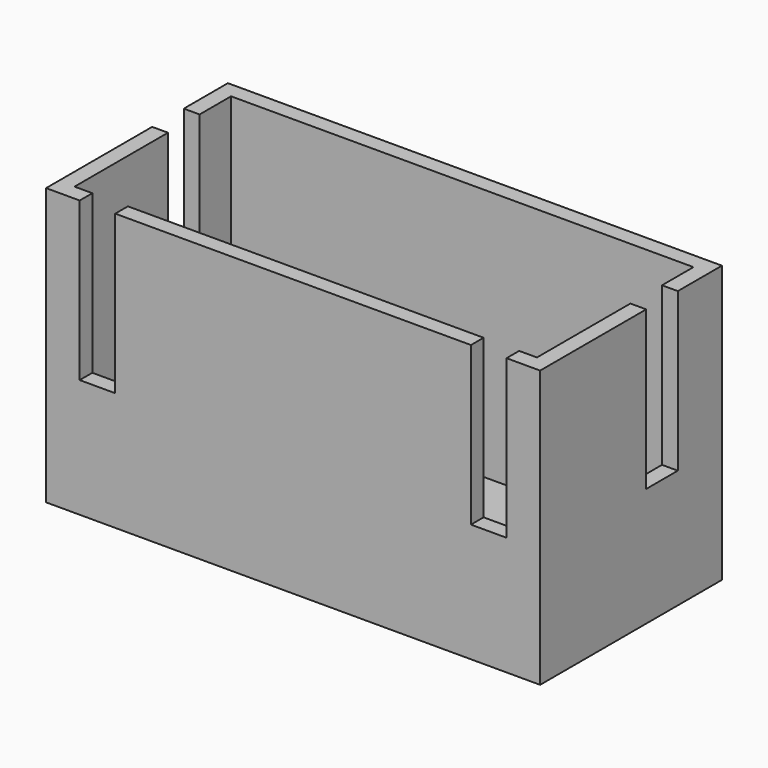
from build123d import *

# Parameters (mm, degrees)
F1_W      = 12.5
F1_H      = 5.75
F2_DEPTH  = 7
F3_W      = 11.7
F3_H      = 4.95
F4_DEPTH  = 6.4
F5_W      = 0.64
F5_H      = 0.64
F6_DEPTH  = 0.601
F7_W      = 0.9
F7_H      = 0.4
F8_DEPTH  = 4
F9_W      = 0.4
F9_H      = 1
F10_DEPTH = 4


# Not quite as in the source:
# - a feature names something its author has since deleted; it is built from what else it names


with BuildPart() as f2:
    # F1 (on Top) → F2 (new body)
    with BuildSketch(Plane.XY):
        with Locations((0, 0.32)):
            Rectangle(F1_W, F1_H)
    extrude(amount=F2_DEPTH)

    # F3 (on face) → F4 (cut)
    with BuildSketch(Plane.XY.offset(7)):
        with Locations((0, 0.32)):
            Rectangle(F3_W, F3_H)
    extrude(amount=-F4_DEPTH, mode=Mode.SUBTRACT)

    # F5 (on face) → F6 (cut, through all)
    with BuildSketch(Plane.XY.offset(0.6)):
        with Locations((-1.25, 0)):
            Rectangle(F5_W, F5_H)
        with Locations((-3.75, 0)):
            Rectangle(F5_W, F5_H)
        with Locations((1.25, 0)):
            Rectangle(F5_W, F5_H)
        with Locations((3.75, 0)):
            Rectangle(F5_W, F5_H)
    extrude(amount=-F6_DEPTH, mode=Mode.SUBTRACT)

    # F7 (on face) → F8 (cut)
    with BuildSketch(Plane.XY.offset(7)):
        with Locations((-4.95, -2.355)):
            Rectangle(F7_W, F7_H)
        with Locations((4.95, -2.355)):
            Rectangle(F7_W, F7_H)
    extrude(amount=-F8_DEPTH, mode=Mode.SUBTRACT)

    # F9 (on face) → F10 (cut)
    with BuildSketch(Plane.XY.offset(7)):
        with Locations((-6.05, 1.3)):
            Rectangle(F9_W, F9_H)
        with Locations((6.05, 1.3)):
            Rectangle(F9_W, F9_H)
    extrude(amount=-F10_DEPTH, mode=Mode.SUBTRACT)


solid = f2.part
